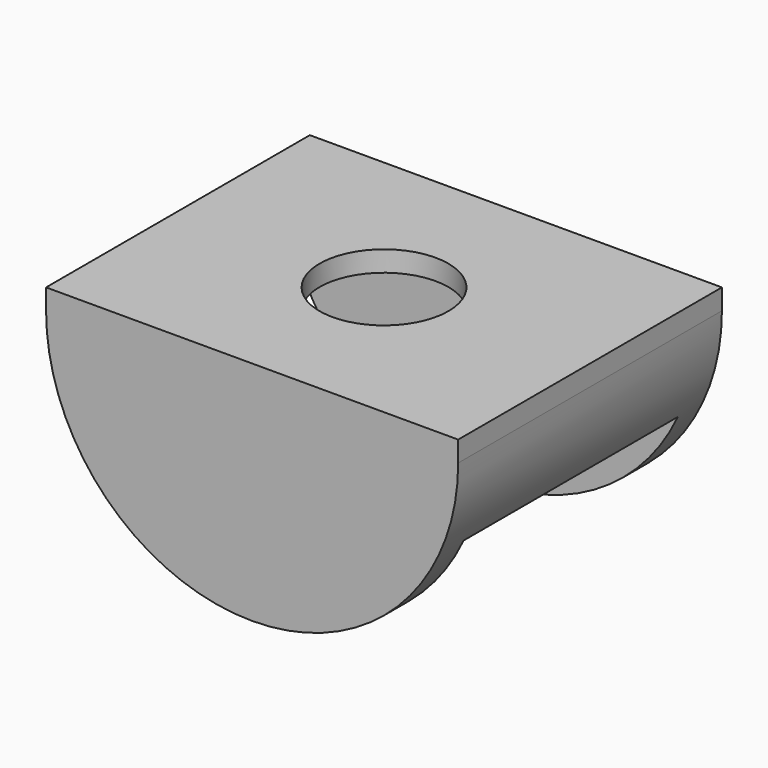
from build123d import *

# Parameters (mm, degrees)
F0_W     = 40
F0_H     = 32
F0_R     = 6.25
F1_DEPTH = 2
F3_START = 13
F3_DEPTH = 3
F4_START = -13
F4_DEPTH = 3
F5_DEPTH = 16


with BuildPart() as f1:
    # F0 (on Top) → F1 (new body)
    with BuildSketch(Plane.XY):
        Rectangle(F0_W, F0_H)
        Circle(F0_R, mode=Mode.SUBTRACT)
    extrude(amount=F1_DEPTH)

    # F2 (on Front) → F3 (join)
    with BuildSketch(Plane.XZ.offset(F3_START)):
        with BuildLine():
            ThreePointArc((18.1261557407, -8.4523652348), (19.5259201424, -4.3287922788), (20, 0))
            Line((20, 0), (18.5, 0))
            ThreePointArc((18.5, 0), (18.0614761317, -4.0041328579), (16.7666940602, -7.8184378422))
            Line((16.7666940602, -7.8184378422), (18.1261557407, -8.4523652348))
        make_face()
        with BuildLine():
            Line((-18.5, 0), (-20, 0))
            ThreePointArc((-20, 0), (-19.5259201424, -4.3287922788), (-18.1261557407, -8.4523652348))
            Line((-18.1261557407, -8.4523652348), (-16.7666940602, -7.8184378422))
            ThreePointArc((-16.7666940602, -7.8184378422), (-18.0614761317, -4.0041328579), (-18.5, 0))
        make_face()
        with BuildLine():
            ThreePointArc((-18.1261557407, -8.4523652348), (0, -20), (18.1261557407, -8.4523652348))
            Line((18.1261557407, -8.4523652348), (16.7666940602, -7.8184378422))
            ThreePointArc((16.7666940602, -7.8184378422), (0, -18.5), (-16.7666940602, -7.8184378422))
            Line((-16.7666940602, -7.8184378422), (-18.1261557407, -8.4523652348))
        make_face()
        with BuildLine():
            ThreePointArc((16.7666940602, -7.8184378422), (18.0614761317, -4.0041328579), (18.5, 0))
            Line((18.5, 0), (0, 0))
            Line((0, 0), (16.7666940602, -7.8184378422))
        make_face()
        with BuildLine():
            Line((0, 0), (-18.5, 0))
            ThreePointArc((-18.5, 0), (-18.0614761317, -4.0041328579), (-16.7666940602, -7.8184378422))
            Line((-16.7666940602, -7.8184378422), (0, 0))
        make_face()
        with BuildLine():
            ThreePointArc((-16.7666940602, -7.8184378422), (0, -18.5), (16.7666940602, -7.8184378422))
            Line((16.7666940602, -7.8184378422), (0, 0))
            Line((0, 0), (-16.7666940602, -7.8184378422))
        make_face()
    extrude(amount=F3_DEPTH)

    # F2 (on Front) → F4 (join)
    with BuildSketch(Plane.XZ.offset(F4_START)):
        with BuildLine():
            ThreePointArc((18.1261557407, -8.4523652348), (19.5259201424, -4.3287922788), (20, 0))
            Line((20, 0), (18.5, 0))
            ThreePointArc((18.5, 0), (18.0614761317, -4.0041328579), (16.7666940602, -7.8184378422))
            Line((16.7666940602, -7.8184378422), (18.1261557407, -8.4523652348))
        make_face()
        with BuildLine():
            Line((-18.5, 0), (-20, 0))
            ThreePointArc((-20, 0), (-19.5259201424, -4.3287922788), (-18.1261557407, -8.4523652348))
            Line((-18.1261557407, -8.4523652348), (-16.7666940602, -7.8184378422))
            ThreePointArc((-16.7666940602, -7.8184378422), (-18.0614761317, -4.0041328579), (-18.5, 0))
        make_face()
        with BuildLine():
            ThreePointArc((-18.1261557407, -8.4523652348), (0, -20), (18.1261557407, -8.4523652348))
            Line((18.1261557407, -8.4523652348), (16.7666940602, -7.8184378422))
            ThreePointArc((16.7666940602, -7.8184378422), (0, -18.5), (-16.7666940602, -7.8184378422))
            Line((-16.7666940602, -7.8184378422), (-18.1261557407, -8.4523652348))
        make_face()
        with BuildLine():
            ThreePointArc((16.7666940602, -7.8184378422), (18.0614761317, -4.0041328579), (18.5, 0))
            Line((18.5, 0), (0, 0))
            Line((0, 0), (16.7666940602, -7.8184378422))
        make_face()
        with BuildLine():
            Line((0, 0), (-18.5, 0))
            ThreePointArc((-18.5, 0), (-18.0614761317, -4.0041328579), (-16.7666940602, -7.8184378422))
            Line((-16.7666940602, -7.8184378422), (0, 0))
        make_face()
        with BuildLine():
            ThreePointArc((-16.7666940602, -7.8184378422), (0, -18.5), (16.7666940602, -7.8184378422))
            Line((16.7666940602, -7.8184378422), (0, 0))
            Line((0, 0), (-16.7666940602, -7.8184378422))
        make_face()
    extrude(amount=-F4_DEPTH)

    # F2 (on Front) → F5 (join, symmetric)
    with BuildSketch(Plane.XZ):
        with BuildLine():
            ThreePointArc((18.1261557407, -8.4523652348), (19.5259201424, -4.3287922788), (20, 0))
            Line((20, 0), (18.5, 0))
            ThreePointArc((18.5, 0), (18.0614761317, -4.0041328579), (16.7666940602, -7.8184378422))
            Line((16.7666940602, -7.8184378422), (18.1261557407, -8.4523652348))
        make_face()
        with BuildLine():
            Line((-18.5, 0), (-20, 0))
            ThreePointArc((-20, 0), (-19.5259201424, -4.3287922788), (-18.1261557407, -8.4523652348))
            Line((-18.1261557407, -8.4523652348), (-16.7666940602, -7.8184378422))
            ThreePointArc((-16.7666940602, -7.8184378422), (-18.0614761317, -4.0041328579), (-18.5, 0))
        make_face()
    extrude(amount=F5_DEPTH, both=True)


solid = f1.part
